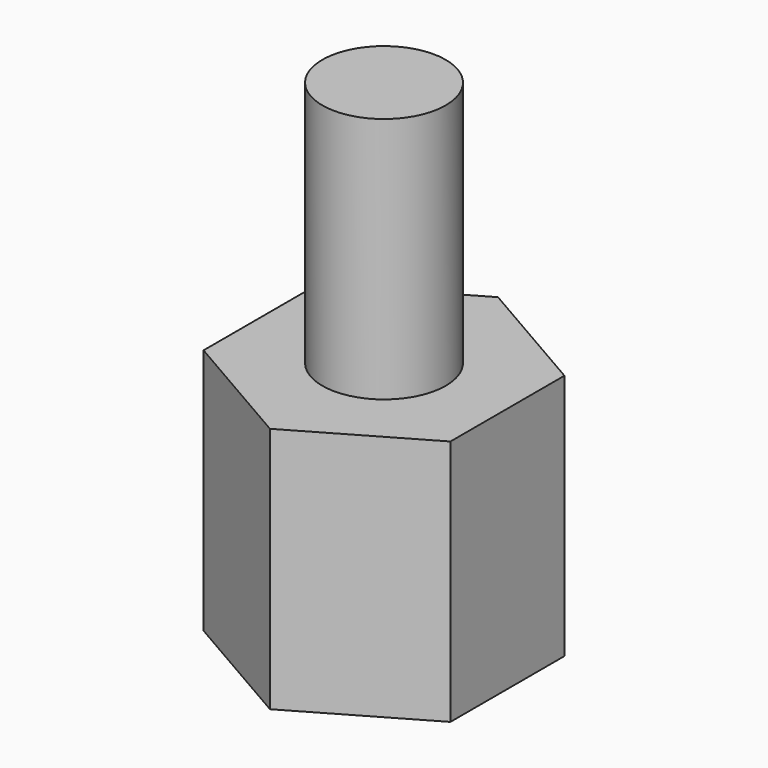
from build123d import *

# Parameters (mm, degrees)
F0_R     = 1
F1_DEPTH = 4
F2_START = 3
F2_DEPTH = 5


with BuildPart() as f1:
    # F0 (on Top) → F1 (new body)
    with BuildSketch(Plane.XY):
        Polygon((-2, 1.1547005384), (-2, -1.1547005384), (0, -2.3094010768), (2, -1.1547005384), (2, 1.1547005384), (0, 2.3094010768), align=None)
        Circle(F0_R, mode=Mode.SUBTRACT)
    extrude(amount=F1_DEPTH)

    # F0 (on Top) → F2 (join)
    with BuildSketch(Plane.XY.offset(F2_START)):
        Circle(F0_R)
    extrude(amount=F2_DEPTH)


solid = f1.part
